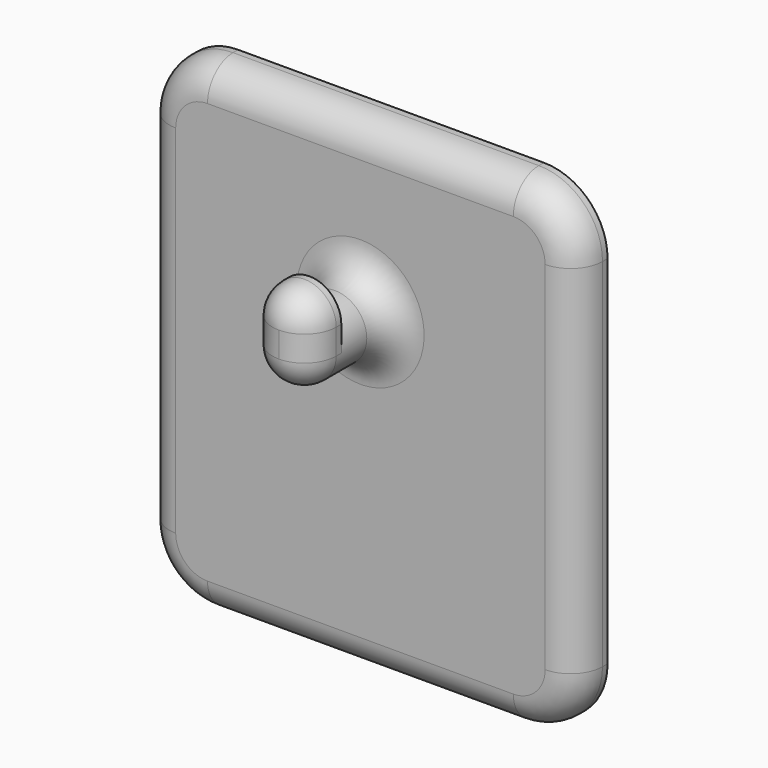
from build123d import *

# Parameters (mm, degrees)
F1_DEPTH     = 3
F3_DEPTH     = 5
F5_DEPTH     = 3
F6_T3_DEPTH  = 28
F6_T5_DEPTH  = 24
F6_T7_DEPTH  = 2
F6_T10_ANGLE = 180
F6_T12_ANGLE = 90
F6_T14_ANGLE = 90
F6_T16_ANGLE = 90
F6_T18_ANGLE = 90
F6_T20_ANGLE = 180


# Not quite as in the source:
# - a fillet or chamfer that OpenCascade refuses, or shapes differently, is made with other operations: its cross-section is extruded or revolved along the edge and cut away or added


with BuildPart() as f1:
    # F0 (on Front) → F1 (new body)
    with BuildSketch(Plane.XZ):
        with BuildLine():
            Line((29, 13), (5, 13))
            ThreePointArc((5, 13), (1.4644660941, 11.5355339059), (0, 8))
            Line((0, 8), (0, -20))
            ThreePointArc((0, -20), (1.4644660941, -23.5355339059), (5, -25))
            Line((5, -25), (29, -25))
            ThreePointArc((29, -25), (32.5355339059, -23.5355339059), (34, -20))
            Line((34, -20), (34, 8))
            ThreePointArc((34, 8), (32.5355339059, 11.5355339059), (29, 13))
        make_face()
    extrude(amount=F1_DEPTH)

    # F2 (on face) → F3 (join)
    with BuildSketch(Plane.XZ.offset(3)):
        with BuildLine():
            ThreePointArc((14.5, 0), (17, -2.5), (19.5, 0))
            ThreePointArc((19.5, 0), (17, 2.5), (14.5, 0))
        make_face()
    extrude(amount=F3_DEPTH)

    # F4 (on face) → F5 (join)
    with BuildSketch(Plane.XZ.offset(8)):
        with BuildLine():
            Line((19.5, 0), (19.5, 2))
            ThreePointArc((19.5, 2), (17, 4.5), (14.5, 2))
            Line((14.5, 2), (14.5, 0))
            ThreePointArc((14.5, 0), (17, -2.5), (19.5, 0))
        make_face()
    extrude(amount=F5_DEPTH)

    # F6: fillet of radius 2.5 on 13 edges, made by hand

    # F6_s1 → F6_t2 (revolve)
    with BuildSketch(Plane.XY):
        with BuildLine():
            ThreePointArc((12, -3), (13.767766953, -3.732233047), (14.5, -5.5))
            Line((14.5, -5.5), (14.5, -3))
            Line((14.5, -3), (12, -3))
        make_face()
    revolve(axis=Axis((17, -3, 0), (0, -1, 0)))

    # F6_s4 → F6_t3 (cut)
    with BuildSketch(Plane.XY.offset(-20)):
        with BuildLine():
            ThreePointArc((34, -0.5), (33.267766953, -2.267766953), (31.5, -3))
            Line((31.5, -3), (34, -3))
            Line((34, -3), (34, -0.5))
        make_face()
        with BuildLine():
            ThreePointArc((2.5, -3), (0.732233047, -2.267766953), (0, -0.5))
            Line((0, -0.5), (0, -3))
            Line((0, -3), (2.5, -3))
        make_face()
    extrude(amount=F6_T3_DEPTH, mode=Mode.SUBTRACT)

    # F6_s6 → F6_t5 (cut)
    with BuildSketch(Plane.YZ.offset(5)):
        with BuildLine():
            ThreePointArc((-3, -22.5), (-2.267766953, -24.267766953), (-0.5, -25))
            Line((-0.5, -25), (-3, -25))
            Line((-3, -25), (-3, -22.5))
        make_face()
        with BuildLine():
            ThreePointArc((-3, 10.5), (-2.267766953, 12.267766953), (-0.5, 13))
            Line((-0.5, 13), (-3, 13))
            Line((-3, 13), (-3, 10.5))
        make_face()
    extrude(amount=F6_T5_DEPTH, mode=Mode.SUBTRACT)

    # F6_s8 → F6_t7 (cut)
    with BuildSketch(Plane.XY):
        with BuildLine():
            ThreePointArc((19.5, -8.5), (18.767766953, -10.267766953), (17, -11))
            Line((17, -11), (19.5, -11))
            Line((19.5, -11), (19.5, -8.5))
        make_face()
        with BuildLine():
            ThreePointArc((17, -11), (15.232233047, -10.267766953), (14.5, -8.5))
            Line((14.5, -8.5), (14.5, -11))
            Line((14.5, -11), (17, -11))
        make_face()
    extrude(amount=F6_T7_DEPTH, mode=Mode.SUBTRACT)

    # F6_s9 → F6_t10 (revolve, cut)
    with BuildSketch(Plane.XY):
        with BuildLine():
            ThreePointArc((14.5, -8.5), (15.232233047, -10.267766953), (17, -11))
            Line((17, -11), (14.5, -11))
            Line((14.5, -11), (14.5, -8.5))
        make_face()
    revolve(axis=Axis((17, -11, 0), (0, -1, 0)), revolution_arc=F6_T10_ANGLE, mode=Mode.SUBTRACT)

    # F6_s11 → F6_t12 (revolve, cut)
    with BuildSketch(Plane.YZ.offset(29)):
        with BuildLine():
            ThreePointArc((-0.5, -25), (-2.267766953, -24.267766953), (-3, -22.5))
            Line((-3, -22.5), (-3, -25))
            Line((-3, -25), (-0.5, -25))
        make_face()
    revolve(axis=Axis((29, -3, -20), (0, -1, 0)), revolution_arc=F6_T12_ANGLE, mode=Mode.SUBTRACT)

    # F6_s13 → F6_t14 (revolve, cut)
    with BuildSketch(Plane.XY.offset(8)):
        with BuildLine():
            ThreePointArc((34, -0.5), (33.267766953, -2.267766953), (31.5, -3))
            Line((31.5, -3), (34, -3))
            Line((34, -3), (34, -0.5))
        make_face()
    revolve(axis=Axis((29, -3, 8), (0, -1, 0)), revolution_arc=F6_T14_ANGLE, mode=Mode.SUBTRACT)

    # F6_s15 → F6_t16 (revolve, cut)
    with BuildSketch(Plane.XY.offset(-20)):
        with BuildLine():
            ThreePointArc((2.5, -3), (0.732233047, -2.267766953), (0, -0.5))
            Line((0, -0.5), (0, -3))
            Line((0, -3), (2.5, -3))
        make_face()
    revolve(axis=Axis((5, -3, -20), (0, -1, 0)), revolution_arc=F6_T16_ANGLE, mode=Mode.SUBTRACT)

    # F6_s17 → F6_t18 (revolve, cut)
    with BuildSketch(Plane.YZ.offset(5)):
        with BuildLine():
            ThreePointArc((-3, 10.5), (-2.267766953, 12.267766953), (-0.5, 13))
            Line((-0.5, 13), (-3, 13))
            Line((-3, 13), (-3, 10.5))
        make_face()
    revolve(axis=Axis((5, -3, 8), (0, -1, 0)), revolution_arc=F6_T18_ANGLE, mode=Mode.SUBTRACT)

    # F6_s19 → F6_t20 (revolve, cut)
    with BuildSketch(Plane.XY.offset(2)):
        with BuildLine():
            ThreePointArc((17, -11), (18.767766953, -10.267766953), (19.5, -8.5))
            Line((19.5, -8.5), (19.5, -11))
            Line((19.5, -11), (17, -11))
        make_face()
    revolve(axis=Axis((17, -11, 2), (0, -1, 0)), revolution_arc=F6_T20_ANGLE, mode=Mode.SUBTRACT)


solid = f1.part
